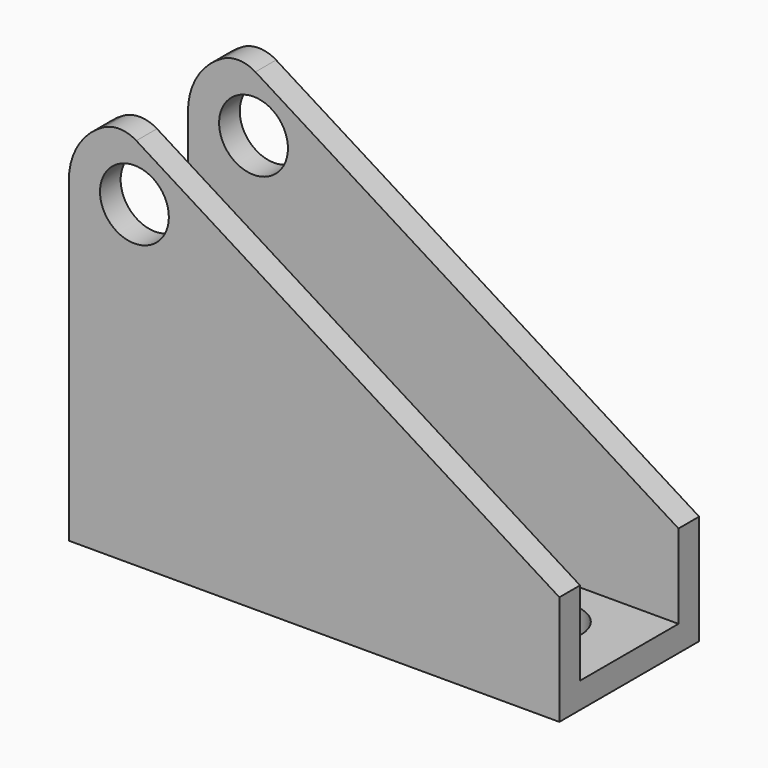
from build123d import *

# Parameters (mm, degrees)
F0_W        = 57
F0_H        = 20.3
F1_DEPTH    = 44.5
F2_W        = 57
F2_H        = 14.3
F3_DEPTH    = 41.5
F4_R        = 7.62
F5_T1_DEPTH = 265.7262717185
F7_R        = 4
F8_DEPTH    = 25.4
F10_D       = 8
F12_D       = 8
F14_DEPTH   = 25.4
F15_R       = 3.81


# Not quite as in the source:
# - a fillet or chamfer that OpenCascade refuses, or shapes differently, is made with other operations: its cross-section is extruded or revolved along the edge and cut away or added
# - a feature of the source that left no trace in its solid (it failed there, or was rolled back) is left out


with BuildPart() as f1:
    # F0 (on Top) → F1 (new body)
    with BuildSketch(Plane.XY):
        with Locations((0.0714529306, -15.5075108656)):
            Rectangle(F0_W, F0_H)
    extrude(amount=F1_DEPTH)

    # F2 (on face) → F3 (cut)
    with BuildSketch(Plane.XY.offset(44.5)):
        with Locations((0.0714529306, -15.5075108656)):
            Rectangle(F2_W, F2_H)
    extrude(amount=-F3_DEPTH, mode=Mode.SUBTRACT)

    # F4
    f4_edges = [f1.edges().sort_by_distance(p)[0] for p in [
        (-28.428547, -24.157511, 44.5),
        (-28.428547, -6.857511, 44.5),
    ]]
    fillet(f4_edges, radius=F4_R)

    # F5: chamfer of 31.75 x 50.8106212971 on 1 edges, made by hand

    # F5_s2 → F5_t1 (cut)
    with BuildSketch(Plane.XZ.offset(-108.7056249936)):
        Polygon((28.5714529306, 12.75), (-22.2391683665, 44.5), (28.5714529306, 44.5), align=None)
    extrude(amount=F5_T1_DEPTH, mode=Mode.SUBTRACT)

    # F7 (on face) → F8 (cut)
    with BuildSketch(Plane.XZ.offset(25.6575108656)):
        with Locations((-20.8085470694, 36.88)):
            Circle(F7_R)
    extrude(amount=-F8_DEPTH, mode=Mode.SUBTRACT)

    # F10 (through all)
    with Locations(Plane.XY.offset(3)):
        with Locations((18.9828891307, -15.5075108656)):
            Hole(F10_D / 2)

    # F12 (through all)
    with Locations(Plane.XY.offset(3)):
        with Locations((-13.3028933778, -15.5075108656)):
            Hole(F12_D / 2)

    # F13 (on face) → F14 (cut)
    with BuildSketch(Plane.XY.offset(3)):
        with BuildLine():
            Line((-28.4285470694, -19.4970791591), (-13.5915884278, -19.4970791591))
            ThreePointArc((-13.5915884278, -19.4970791591), (-17.3028933778, -15.5075108656), (-13.5915884278, -11.5179425722))
            Line((-13.5915884278, -11.5179425722), (-13.5915884278, -11.4970791591))
            Line((-13.5915884278, -11.4970791591), (-28.4285470694, -11.4970791591))
            Line((-28.4285470694, -11.4970791591), (-28.4285470694, -19.4970791591))
        make_face()
    extrude(amount=-F14_DEPTH, mode=Mode.SUBTRACT)

    # F15
    f15_edges = [f1.edges().sort_by_distance(p)[0] for p in [
        (-22.070718, -24.157511, 44.39474),
        (-22.070718, -6.857511, 44.39474),
    ]]
    fillet(f15_edges, radius=F15_R)


solid = f1.part
